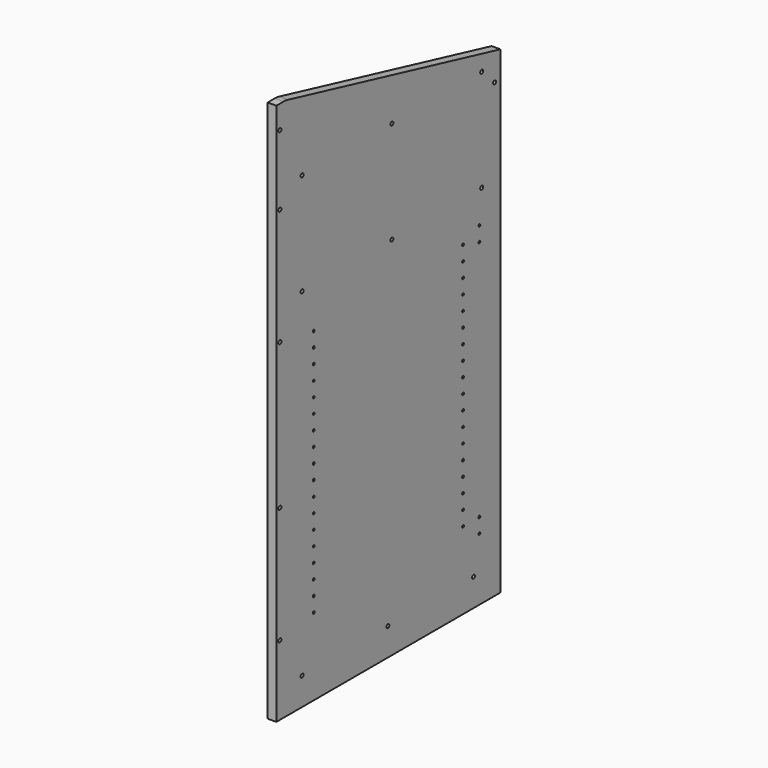
from build123d import *

# Parameters (mm, degrees)
F1_DEPTH = 19.05
F3_D     = 8.001
F3_DEPTH = 14.224
F3_TIP   = 2.4037429064
F5_D     = 5.0038
F5_DEPTH = 14.224
F5_TIP   = 1.5032931827
F9_D     = 5.0038
F9_DEPTH = 14.224
F9_TIP   = 1.5032931827


# Not quite as in the source:
# - a feature names something its author has since deleted; it is built from what else it names


with BuildPart() as f1:
    # F0 (on Right) → F1 (new body)
    with BuildSketch(Plane.YZ):
        with BuildLine():
            Line((304.8, -590.55), (304.8, 590.55))
            Line((304.8, 590.55), (285.3894786878, 590.55))
            ThreePointArc((285.3894786878, 590.55), (279.4412012464, 590.2005500018), (273.5747594562, 589.157007696))
            Line((273.5747594562, 589.157007696), (-304.8, 450.85))
            Line((-304.8, 450.85), (-304.8, 428.625))
            Line((-304.8, 428.625), (-304.8, -590.55))
            Line((-304.8, -590.55), (304.8, -590.55))
        make_face()
    extrude(amount=F1_DEPTH)

    # F3
    with Locations(Plane.YZ.offset(19.05)):
        with Locations((-254, 428.625), (-288.925, 393.7), (-9.525, 428.625), (234.95, 428.625), (-254, 206.375), (-9.525, 206.375), (234.95, 206.375), (295.0947393439, 539.75), (295.0947393439, 387.35), (295.0947393439, 133.35), (295.275, -184.15), (295.275, -438.15), (234.95, -530.225), (-231.775, -530.225), (1.397, -530.225)):
            Hole(F3_D / 2, depth=F3_DEPTH)
            with Locations((0, 0, -(F3_DEPTH + F3_TIP / 2))):  # 118° drill point
                Cone(0, F3_D / 2, F3_TIP, mode=Mode.SUBTRACT)

    # F5
    with Locations(Plane.YZ.offset(19.05)):
        with Locations((-203.2, 117.475), (-203.2, 85.725), (-203.2, 53.975), (-203.2, 22.225), (-203.2, -9.525), (-203.2, -41.275), (-203.2, -73.025), (-203.2, -104.775), (-203.2, -136.525), (-203.2, -168.275), (-203.2, -200.025), (-203.2, -231.775), (-203.2, -263.525), (-203.2, -295.275), (-203.2, -327.025), (-203.2, -358.775), (-203.2, -390.525), (-203.2, -422.275), (203.2, -422.275), (203.2, -390.525), (203.2, -358.775), (203.2, -327.025), (203.2, -295.275), (203.2, -263.525), (203.2, -231.775), (203.2, -200.025), (203.2, -168.275), (203.2, -136.525), (203.2, -104.775), (203.2, -73.025), (203.2, -41.275), (203.2, -9.525), (203.2, 22.225), (203.2, 53.975), (203.2, 85.725), (203.2, 117.475)):
            Hole(F5_D / 2, depth=F5_DEPTH)
            with Locations((0, 0, -(F5_DEPTH + F5_TIP / 2))):  # 118° drill point
                Cone(0, F5_D / 2, F5_TIP, mode=Mode.SUBTRACT)


with BuildPart() as f6_1:
    # F6: instance of F1
    add(f1.part.mirror(Plane(origin=(9.525, 304.8, 0), x_dir=(-1, 0, 0), z_dir=(0, 1, 0))))

    # F9
    with Locations(Plane.YZ.offset(19.05)):
        with Locations((857.25, 136.525), (857.25, 104.775), (857.25, -422.275), (857.25, -454.025)):
            Hole(F9_D / 2, depth=F9_DEPTH)
            with Locations((0, 0, -(F9_DEPTH + F9_TIP / 2))):  # 118° drill point
                Cone(0, F9_D / 2, F9_TIP, mode=Mode.SUBTRACT)


solid = f6_1.part
